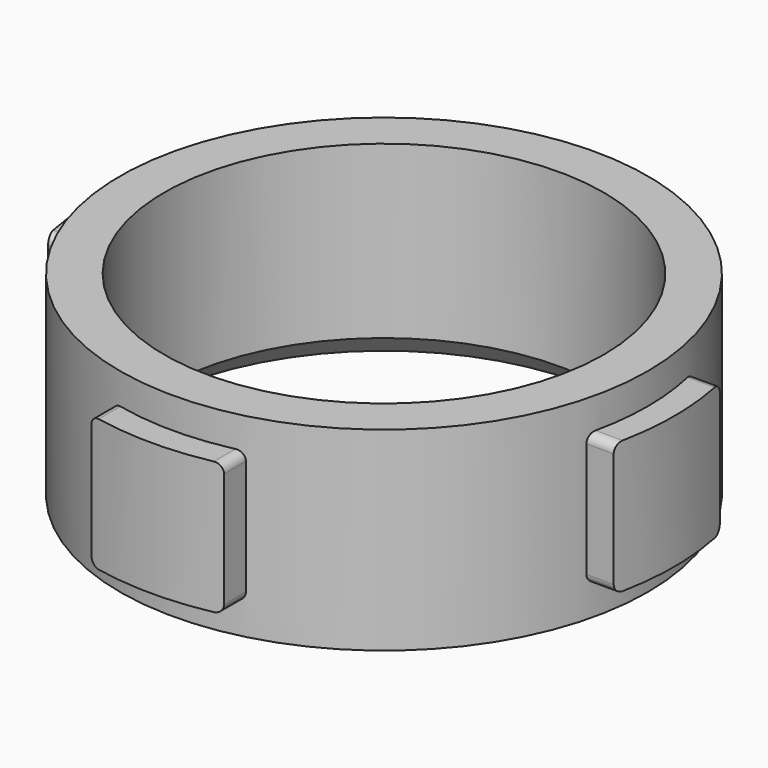
from build123d import *

# Parameters (mm, degrees)
F3_DEPTH        = 38.3
F3_COPIES_COUNT = 4
F4_R            = 24.85
F5_DEPTH        = 25
F6_R            = 51.6597982195
F6_R_2          = 32.85
F7_DEPTH        = 25


# Not quite as in the source:
# - a pattern or mirror of a feature is missing from the dataset's text; its kind, count and spacing are read off the source's solid


with BuildPart() as f1:
    # F0 (on Front) → F1 (revolve)
    with BuildSketch(Plane.XZ):
        Polygon((29.85, 0), (24.85, 0), (24.85, -19.35), (27.5, -22), (29.85, -22), align=None)
    revolve(axis=Axis((0, 0, -5.2975), (0, 0, -1)))

    # F2 (on Front) → F3 (join)
    with BuildSketch(Plane.XZ):
        with BuildLine():
            ThreePointArc((-7.5, -17.5), (-7.2071067812, -18.2071067812), (-6.5, -18.5))
            Line((-6.5, -18.5), (6.5, -18.5))
            ThreePointArc((6.5, -18.5), (7.2071067812, -18.2071067812), (7.5, -17.5))
            Line((7.5, -17.5), (7.5, -4.5))
            ThreePointArc((7.5, -4.5), (7.2071067812, -3.7928932188), (6.5, -3.5))
            Line((6.5, -3.5), (-6.5, -3.5))
            ThreePointArc((-6.5, -3.5), (-7.2071067812, -3.7928932188), (-7.5, -4.5))
            Line((-7.5, -4.5), (-7.5, -17.5))
        make_face()
    f3 = extrude(amount=F3_DEPTH)

    # F3_copies: F3 ×4 about axis
    f3_copies_axis = Axis((0, 0, 0), (0, 0, 1))
    for i in range(1, F3_COPIES_COUNT):
        add(f3.rotate(f3_copies_axis, i * 360 / F3_COPIES_COUNT))

    # F4 (on face) → F5 (cut)
    with BuildSketch(Plane.XY):
        Circle(F4_R)
    extrude(amount=-F5_DEPTH, mode=Mode.SUBTRACT)

    # F6 (on face) → F7 (cut)
    with BuildSketch(Plane.XY):
        Circle(F6_R)
        Circle(F6_R_2, mode=Mode.SUBTRACT)
    extrude(amount=-F7_DEPTH, mode=Mode.SUBTRACT)


solid = f1.part
